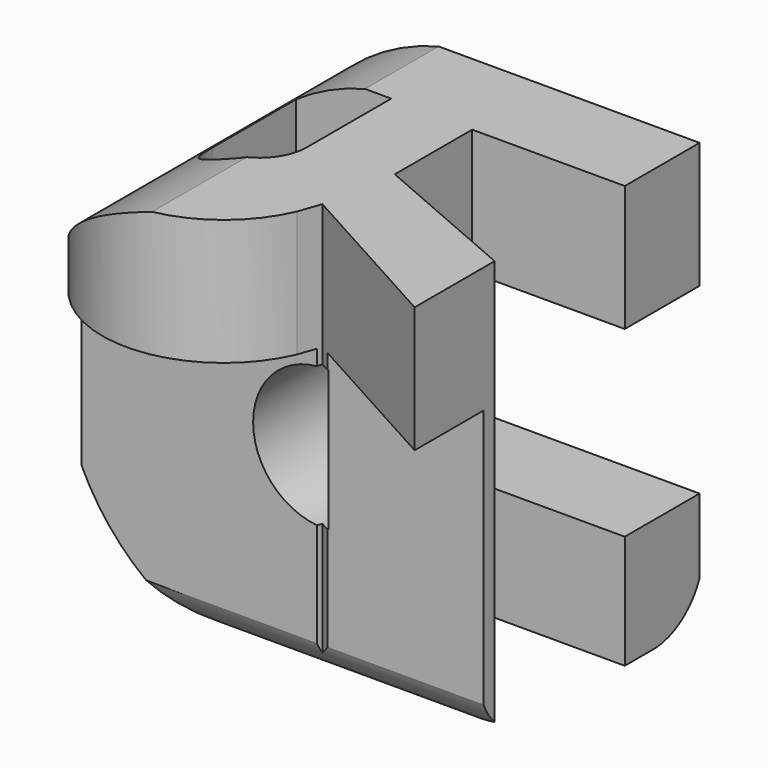
from build123d import *

# Parameters (mm, degrees)
F0_W     = 50
F0_H     = 50
F1_DEPTH = 50
F3_DEPTH = 50.001
F5_DEPTH = 50.001
F7_DEPTH = 50.001


# Not quite as in the source:
# - a feature names something its author has since deleted; it is built from what else it names


with BuildPart() as f1:
    # F0 (on Top) → F1 (new body)
    with BuildSketch(Plane.XY):
        Rectangle(F0_W, F0_H)
    extrude(amount=F1_DEPTH)

    # F2 (on face) → F3 (cut, through all)
    with BuildSketch(Plane(origin=(0, 25, 0), x_dir=(-1, 0, 0), z_dir=(0, 1, 0))):
        with BuildLine():
            ThreePointArc((-6.6122752614, 16.6977748275), (2.2958755953, 25), (-6.6122752614, 33.3022251725))
            Line((-6.6122752614, 33.3022251725), (-6.6122752614, 16.6977748275))
        make_face()
        with BuildLine():
            ThreePointArc((5.8814799413, 50), (19.5641723767, 41.0564068722), (25, 25.640320846))
            Line((25, 25.640320846), (25, 50))
            Line((25, 50), (5.8814799413, 50))
        make_face()
        with BuildLine():
            Line((25, 0), (25, 24.359679154))
            ThreePointArc((25, 24.359679154), (19.5641723767, 8.9435931278), (5.8814799413, 0))
            Line((5.8814799413, 0), (25, 0))
        make_face()
    extrude(amount=-F3_DEPTH, mode=Mode.SUBTRACT)

    # F4 (on face) → F5 (cut, through all)
    with BuildSketch(Plane.YZ.offset(25)):
        Polygon((-6.9390782155, 35.097297281), (-25, 35.097297281), (-25, 0), (-6.9390782155, 0), (-6.9390782155, 4.401256796), (-6.9390782155, 13.4532200173), align=None)
        with BuildLine():
            Line((25, 13.4532200173), (25, 35.097297281))
            Line((25, 35.097297281), (6.9390782155, 35.097297281))
            Line((6.9390782155, 35.097297281), (6.9390782155, 13.4532200173))
            ThreePointArc((6.9390782155, 13.4532200173), (10.1754756179, 10.2168226149), (13.4118730202, 13.4532200173))
            Line((13.4118730202, 13.4532200173), (25, 13.4532200173))
        make_face()
        with BuildLine():
            Line((25, 0), (25, 4.6294564381))
            ThreePointArc((25, 4.6294564381), (22.4439231862, 1.4056456338), (18.5773167759, 0))
            Line((18.5773167759, 0), (25, 0))
        make_face()
        with BuildLine():
            Line((-6.9390782155, 4.401256796), (-6.9390782155, 0))
            Line((-6.9390782155, 0), (-1.2912911565, 0))
            ThreePointArc((-1.2912911565, 0), (-4.7087911569, 1.438899851), (-6.9390782155, 4.401256796))
        make_face()
    extrude(amount=-F5_DEPTH, mode=Mode.SUBTRACT)

    # F6 (on face) → F7 (cut, through all)
    with BuildSketch(Plane(origin=(0, 0, 0), x_dir=(1, 0, 0), z_dir=(0, 0, -1))):
        Polygon((-27.4569652975, -12.0541369542), (-23.0521892468, -12.0541369542), (-23.0521892468, 3.30411084), (-23.0521892468, 9.0968515724), (-27.4569652975, 9.0968515724), align=None)
        Polygon((6.9360537454, -13.9329824597), (25, -13.9329824597), (25, 1.2912911565), (15.6700833973, 1.2912911565), (6.9360537454, -2.4867046159), align=None)
        with BuildLine():
            Line((-23.0521892468, 9.0968515724), (-23.0521892468, 3.30411084))
            ThreePointArc((-23.0521892468, 3.30411084), (-11.5730780457, 17.3836701729), (4.5299022458, 8.9754592627))
            Line((4.5299022458, 8.9754592627), (5.442249123, 6.361215841))
            Line((5.442249123, 6.361215841), (25, 17.1625725925))
            Line((25, 17.1625725925), (25, 25))
            Line((25, 25), (-23.0521892468, 25))
            Line((-23.0521892468, 25), (-23.0521892468, 9.0968515724))
        make_face()
        Polygon((15.6700833973, 1.2912911565), (25, 1.2912911565), (25, 5.3270440549), align=None)
        with BuildLine():
            Line((-5.8814799413, 1.2912911565), (-5.8814799413, -14.1096981242))
            Line((-5.8814799413, -14.1096981242), (-2.7823168784, -14.1096981242))
            Line((-2.7823168784, -14.1096981242), (-2.7823168784, -1.6426106449))
            ThreePointArc((-2.7823168784, -1.6426106449), (-2.9925352611, -0.1187433848), (-3.6074871188, 1.2912911565))
            Line((-3.6074871188, 1.2912911565), (-5.8814799413, 1.2912911565))
        make_face()
        with BuildLine():
            Line((-14.0390070155, -14.1096981242), (-5.8814799413, -14.1096981242))
            Line((-5.8814799413, -14.1096981242), (-5.8814799413, 1.2912911565))
            Line((-5.8814799413, 1.2912911565), (-3.6074871188, 1.2912911565))
            ThreePointArc((-3.6074871188, 1.2912911565), (-9.9345292071, 3.7755160409), (-14.0390070155, -1.6426106449))
            Line((-14.0390070155, -1.6426106449), (-14.0390070155, -14.1096981242))
        make_face()
    extrude(amount=-F7_DEPTH, mode=Mode.SUBTRACT)


solid = f1.part
